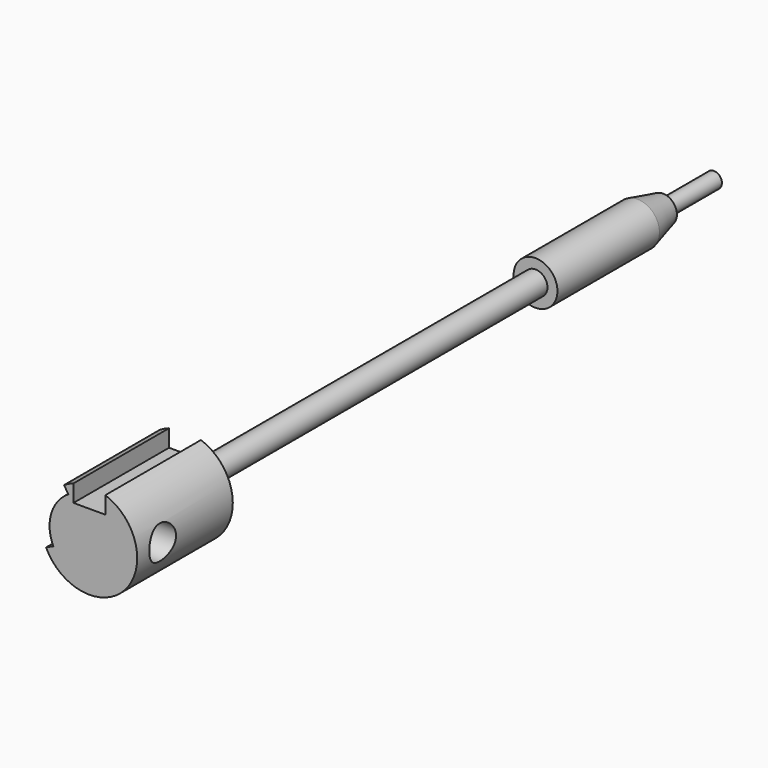
from build123d import *

# Parameters (mm, degrees)
F0_R      = 1
F1_DEPTH  = 8
F2_R      = 2.75
F3_DEPTH  = 80
F4_SIZE2  = 1
F4_SIZE   = 4
F5_R      = 6
F5_R_2    = 2.75
F6_DEPTH  = 5
F7_DEPTH  = 10
F12_R     = 2.75
F12_R_2   = 1.5
F13_DEPTH = 55
F15_D     = 4.2
F16_W     = 4
F16_H     = 15
F17_DEPTH = 2.5
F24_DEPTH = 15


with BuildPart() as f1:
    # F0 (on Front) → F1 (new body)
    with BuildSketch(Plane.XZ):
        Circle(F0_R)
    extrude(amount=-F1_DEPTH)

    # F2 (on face) → F3 (join)
    with BuildSketch(Plane.XZ):
        Circle(F2_R)
    extrude(amount=F3_DEPTH)

    # F4
    f4_edges = [f1.edges().sort_by_distance(p)[0] for p in [
        (-2.75, 0, 0),
    ]]
    f4_side = f1.faces().sort_by_distance((-2.75, -40, 0))[0]
    chamfer(f4_edges, length=F4_SIZE, length2=F4_SIZE2, reference=f4_side)

    # F5 (on face) → F6 (join)
    with BuildSketch(Plane.XZ.offset(80)):
        Circle(F5_R)
        Circle(F5_R_2, mode=Mode.SUBTRACT)
    extrude(amount=-F6_DEPTH)

    # F7 (add): a face of the model
    f7_faces = [f1.faces().sort_by_distance(p)[0] for p in [
        (0, -80, 0),
    ]]
    extrude(f7_faces, amount=F7_DEPTH)

    # F12 (on face) → F13 (cut)
    with BuildSketch(Plane(origin=(0, -75, 0), x_dir=(-1, 0, 0), z_dir=(0, 1, 0))):
        Circle(F12_R)
        Circle(F12_R_2, mode=Mode.SUBTRACT)
    extrude(amount=F13_DEPTH, mode=Mode.SUBTRACT)

    # F15 (through all)
    with Locations(Plane.YZ.offset(6)):
        with Locations((-86, 0)):
            Hole(F15_D / 2)

    # F16 (on offset) → F17 (cut)
    with BuildSketch(Plane.XY.offset(6)):
        with Locations((0, -82.5)):
            Rectangle(F16_W, F16_H)
    extrude(amount=-F17_DEPTH, mode=Mode.SUBTRACT)

    # F23 (on face) → F24 (cut)
    with BuildSketch(Plane.XZ.offset(90)):
        with BuildLine():
            ThreePointArc((-3.1795155854, 5.0882885769), (-5.7529184092, 1.7040920682), (-5.4378467222, -2.5357095704))
            Line((-5.4378467222, -2.5357095704), (-4.5315389352, -2.1130913087))
            ThreePointArc((-4.5315389352, -2.1130913087), (-4.7940986743, 1.4200767235), (-2.6495963212, 4.2402404808))
            Line((-2.6495963212, 4.2402404808), (-3.1795155854, 5.0882885769))
        make_face()
    extrude(amount=-F24_DEPTH, mode=Mode.SUBTRACT)


solid = f1.part
